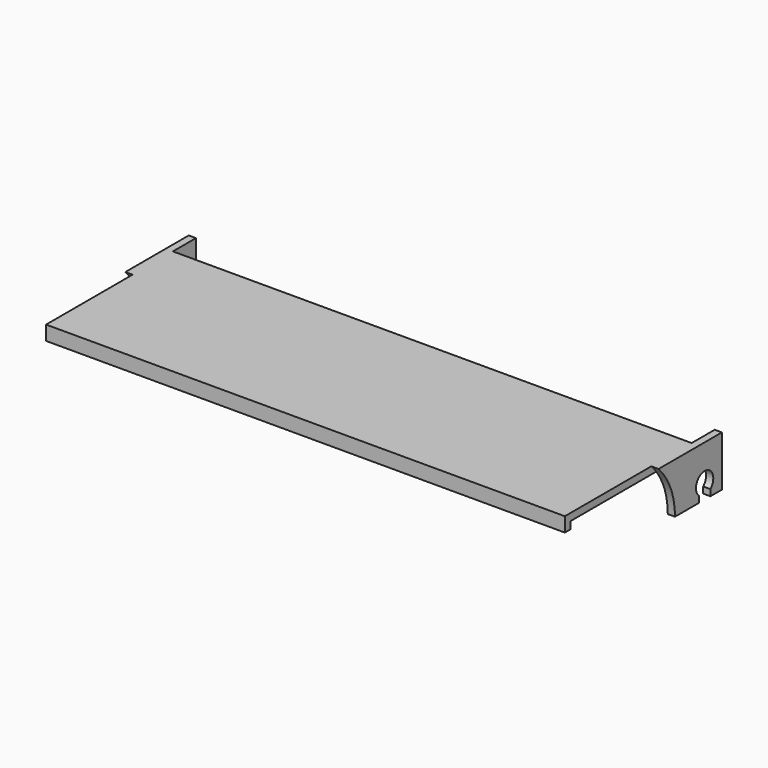
from build123d import *

# Parameters (mm, degrees)
F1_DEPTH = 72
F3_DEPTH = 2
F4_W     = 23
F4_H     = 4
F5_DEPTH = 25


# Not quite as in the source:
# - a pattern or mirror of a feature is missing from the dataset's text; its kind, count and spacing are read off the source's solid


with BuildPart() as f1:
    # F0 (on Right) → F1 (new body, symmetric)
    with BuildSketch(Plane.YZ):
        Polygon((-22, 23), (-20, 23), (-20, 25), (20, 25), (20, 21), (22, 21), (22, 27), (-22, 27), align=None)
    extrude(amount=F1_DEPTH, both=True)

    # F2 (on face) → F3 (join)
    with BuildSketch(Plane.YZ.offset(72)):
        with BuildLine():
            Line((30, 27), (22, 27))
            Line((22, 27), (8, 27))
            ThreePointArc((8, 27), (12.2327735284, 20.5611792354), (13.7171431429, 13))
            Line((13.7171431429, 13), (22, 13))
            Line((22, 13), (22, 14.7639320225))
            ThreePointArc((22, 14.7639320225), (24, 20), (26, 14.7639320225))
            Line((26, 14.7639320225), (26, 13))
            Line((26, 13), (30, 13))
            Line((30, 13), (30, 27))
        make_face()
    f3 = extrude(amount=F3_DEPTH)

    # F3_copies: F3 across plane
    add(f3.mirror(Plane(origin=(0, 0, 0), x_dir=(0, 0, -1), z_dir=(-1, 0, 0))))

    # F4 (on face) → F5 (cut)
    with BuildSketch(Plane(origin=(0, 22, 0), x_dir=(-1, 0, 0), z_dir=(0, 1, 0))):
        with Locations((46.5, 23)):
            Rectangle(F4_W, F4_H)
    extrude(amount=-F5_DEPTH, mode=Mode.SUBTRACT)


solid = f1.part
